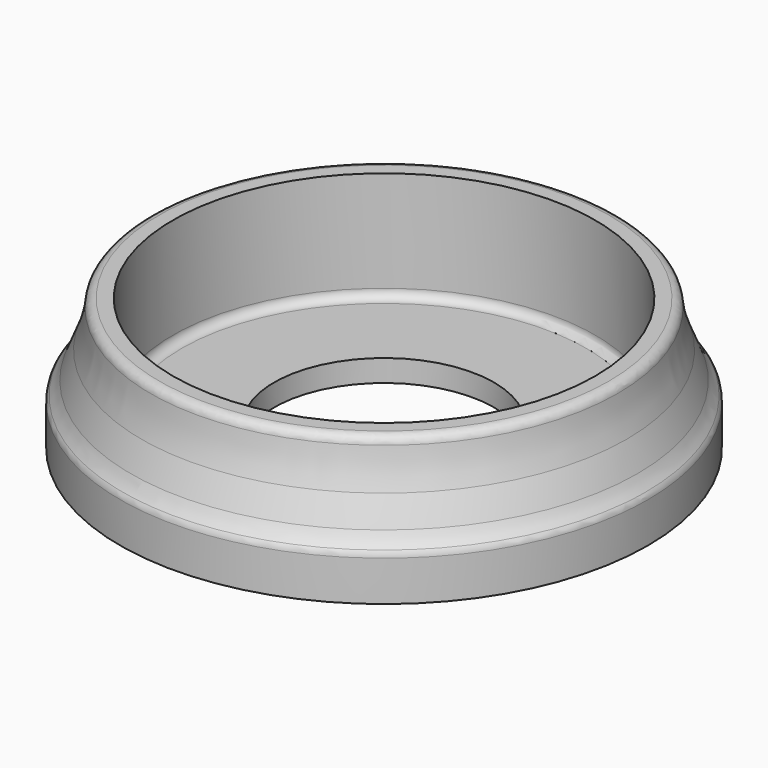
from build123d import *

# Parameters (mm, degrees)
F0_R     = 60
F0_R_2   = 25
F1_DEPTH = 30
F2_R     = 48
F2_R_2   = 25
F3_DEPTH = 25
F4_R     = 2
F5_R     = 60
F5_R_2   = 53
F6_DEPTH = 20
F7_SIZE2 = 6
F7_SIZE  = 15
F10_R    = 2
F11_R    = 2


# Not quite as in the source:
# - a fillet or chamfer that OpenCascade refuses, or shapes differently, is made with other operations: its cross-section is extruded or revolved along the edge and cut away or added


with BuildPart() as f1:
    # F0 (on Top) → F1 (new body)
    with BuildSketch(Plane.XY):
        Circle(F0_R)
        Circle(F0_R_2, mode=Mode.SUBTRACT)
    extrude(amount=F1_DEPTH)

    # F2 (on face) → F3 (cut)
    with BuildSketch(Plane.XY.offset(30)):
        Circle(F2_R)
        Circle(F2_R_2, mode=Mode.SUBTRACT)
    extrude(amount=-F3_DEPTH, mode=Mode.SUBTRACT)

    # F4
    f4_edges = [f1.edges().sort_by_distance(p)[0] for p in [
        (-48, 0, 5),
    ]]
    fillet(f4_edges, radius=F4_R)

    # F5 (on face) → F6 (cut)
    with BuildSketch(Plane.XY.offset(30)):
        Circle(F5_R)
        Circle(F5_R_2, mode=Mode.SUBTRACT)
    extrude(amount=-F6_DEPTH, mode=Mode.SUBTRACT)

    # F7
    f7_edges = [f1.edges().sort_by_distance(p)[0] for p in [
        (-53, 0, 10),
    ]]
    chamfer(f7_edges, length=F7_SIZE, length2=F7_SIZE2)

    # F8: fillet of radius 10 on 1 edges, made by hand

    # F8_s1 → F8_t2 (revolve)
    with BuildSketch(Plane.XZ):
        with BuildLine():
            ThreePointArc((57.575110205, 13.5622244876), (58.5933939753, 11.6489422086), (60, 10))
            Line((60, 10), (59, 10))
            Line((59, 10), (57.575110205, 13.5622244876))
        make_face()
    revolve(axis=Axis((0, 0, 10), (0, 0, 1)))

    # F9: fillet of radius 30 on 1 edges, made by hand

    # F9_s1 → F9_t2 (revolve)
    with BuildSketch(Plane.XZ):
        with BuildLine():
            ThreePointArc((53, 30), (53.6092390565, 24.7367266148), (55.134911926, 19.662720185))
            Line((55.134911926, 19.662720185), (53, 25))
            Line((53, 25), (53, 30))
        make_face()
    revolve(axis=Axis((0, 0, 25), (0, 0, 1)))

    # F10
    f10_edges = [f1.edges().sort_by_distance(p)[0] for p in [
        (-60, 0, 10),
    ]]
    fillet(f10_edges, radius=F10_R)

    # F11
    f11_edges = [f1.edges().sort_by_distance(p)[0] for p in [
        (-53, 0, 30),
    ]]
    fillet(f11_edges, radius=F11_R)


solid = f1.part
